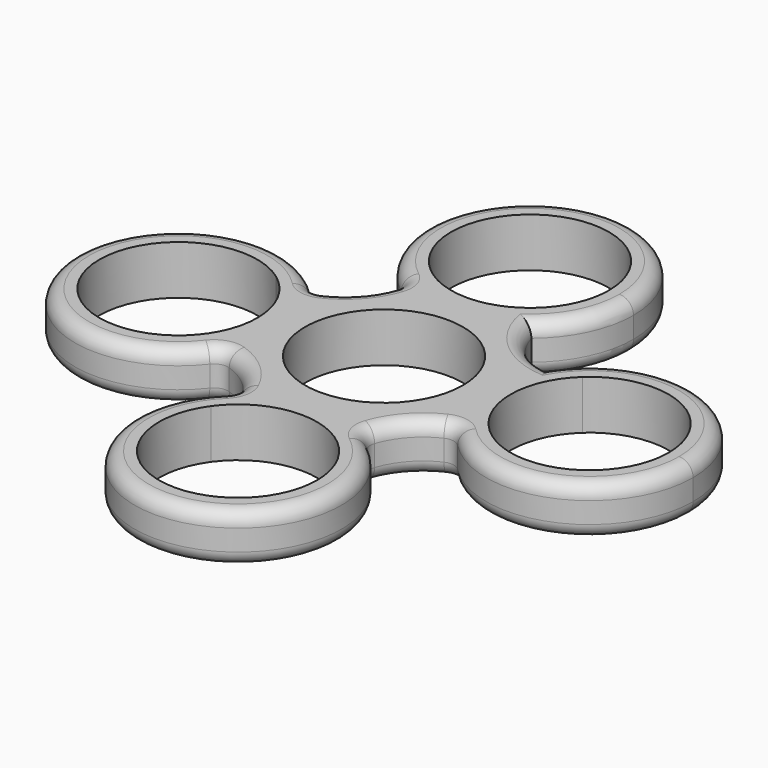
from build123d import *

# Parameters (mm, degrees)
F0_R     = 11.25
F1_DEPTH = 7
F2_R     = 2


with BuildPart() as f1:
    # F0 (on Top) → F1 (new body)
    with BuildSketch(Plane.XY):
        with BuildLine():
            ThreePointArc((-20.6818419333, 15.0335644628), (-21.5385463681, 19.9857387785), (-24.0090837029, 24.3623148626))
            ThreePointArc((-24.0090837029, 24.3623148626), (-26.4040491127, 23.960385675), (-28.8254223349, 24.1457450693))
            ThreePointArc((-28.8254223349, 24.1457450693), (-25.4035315724, 20.1491048046), (-24.1731995815, 15.0335644628))
            ThreePointArc((-24.1731995815, 15.0335644628), (-25.1151928743, 10.5271803553), (-27.7834213991, 6.7754599996))
            ThreePointArc((-27.7834213991, 6.7754599996), (-25.4145244015, 7.2193338549), (-23.0081257396, 7.0853843686))
            ThreePointArc((-23.0081257396, 7.0853843686), (-21.2753610709, 10.8927564753), (-20.6818419333, 15.0335644628))
        make_face()
        with BuildLine():
            ThreePointArc((-28.8254223349, 24.1457450693), (-26.4040491127, 23.960385675), (-24.0090837029, 24.3623148626))
            ThreePointArc((-24.0090837029, 24.3623148626), (-50.1398789796, 14.1809374616), (-23.0081257396, 7.0853843686))
            ThreePointArc((-23.0081257396, 7.0853843686), (-25.4145244015, 7.2193338549), (-27.7834213991, 6.7754599996))
            ThreePointArc((-27.7834213991, 6.7754599996), (-46.6530124471, 14.3599154428), (-28.8254223349, 24.1457450693))
        make_face()
        with BuildLine():
            ThreePointArc((0.2988637144, 33.2261356881), (-8.1772596841, 29.9235721685), (-16.9780667795, 32.2251777247))
            ThreePointArc((-16.9780667795, 32.2251777247), (-19.3767240664, 27.2950515881), (-24.0090837029, 24.3623148626))
            ThreePointArc((-24.0090837029, 24.3623148626), (-21.5385463681, 19.9857387785), (-20.6818419333, 15.0335644628))
            ThreePointArc((-20.6818419333, 15.0335644628), (-21.2753610709, 10.8927564753), (-23.0081257396, 7.0853843686))
            ThreePointArc((-23.0081257396, 7.0853843686), (-18.0779996029, 4.6867270817), (-15.1452628774, 0.0543674452))
            ThreePointArc((-15.1452628774, 0.0543674452), (-6.6691394789, 3.3569309648), (2.1316676166, 1.0553254086))
            ThreePointArc((2.1316676166, 1.0553254086), (4.5303249035, 5.9854515452), (9.16268454, 8.9181882707))
            ThreePointArc((9.16268454, 8.9181882707), (5.8601210204, 17.3943116693), (8.1617265766, 26.1951187647))
            ThreePointArc((8.1617265766, 26.1951187647), (3.23160044, 28.5937760516), (0.2988637144, 33.2261356881))
        make_face()
        with Locations((-7.4231995815, 16.6402515666)):
            Circle(F0_R, mode=Mode.SUBTRACT)
        with BuildLine():
            ThreePointArc((0.0822939211, 38.0424743201), (-8.3562376653, 33.410438701), (-17.2879911485, 37.0004733843))
            ThreePointArc((-17.2879911485, 37.0004733843), (-16.8441172933, 34.6315763866), (-16.9780667795, 32.2251777247))
            ThreePointArc((-16.9780667795, 32.2251777247), (-8.1772596841, 29.9235721685), (0.2988637144, 33.2261356881))
            ThreePointArc((0.2988637144, 33.2261356881), (-0.1030654731, 35.6211010979), (0.0822939211, 38.0424743201))
        make_face()
        with BuildLine():
            ThreePointArc((-17.2879911485, 37.0004733843), (-13.1322533674, 55.1156077709), (2.2201133147, 44.6402515666))
            ThreePointArc((2.2201133147, 44.6402515666), (1.6723217742, 41.1725096373), (0.0822939211, 38.0424743201))
            ThreePointArc((0.0822939211, 38.0424743201), (-0.1030654731, 35.6211010979), (0.2988637144, 33.2261356881))
            ThreePointArc((0.2988637144, 33.2261356881), (4.2897617966, 38.3240351653), (5.7114709628, 44.6402515666))
            ThreePointArc((5.7114709628, 44.6402515666), (-16.1059258277, 57.5722775241), (-16.9780667795, 32.2251777247))
            ThreePointArc((-16.9780667795, 32.2251777247), (-16.8441172933, 34.6315763866), (-17.2879911485, 37.0004733843))
        make_face()
        with BuildLine():
            ThreePointArc((35.3181580667, 18.2469386705), (24.717608406, 32.394777181), (8.1617265766, 26.1951187647))
            ThreePointArc((8.1617265766, 26.1951187647), (10.5681252385, 26.0611692784), (12.9370222362, 26.5050431337))
            ThreePointArc((12.9370222362, 26.5050431337), (25.083184526, 28.5549453777), (31.8268004185, 18.2469386705))
            ThreePointArc((31.8268004185, 18.2469386705), (25.6923407603, 8.2272706614), (13.979023172, 9.134758064))
            ThreePointArc((13.979023172, 9.134758064), (11.5576499498, 9.3201174583), (9.16268454, 8.9181882707))
            ThreePointArc((9.16268454, 8.9181882707), (25.5289747343, 4.3622854571), (35.3181580667, 18.2469386705))
        make_face()
        with BuildLine():
            ThreePointArc((12.9370222362, 26.5050431337), (10.5681252385, 26.0611692784), (8.1617265766, 26.1951187647))
            ThreePointArc((8.1617265766, 26.1951187647), (5.8601210204, 17.3943116693), (9.16268454, 8.9181882707))
            ThreePointArc((9.16268454, 8.9181882707), (11.5576499498, 9.3201174583), (13.979023172, 9.134758064))
            ThreePointArc((13.979023172, 9.134758064), (9.3469875529, 17.5732896505), (12.9370222362, 26.5050431337))
        make_face()
        with BuildLine():
            ThreePointArc((2.1316676166, 1.0553254086), (-6.6691394789, 3.3569309648), (-15.1452628774, 0.0543674452))
            ThreePointArc((-15.1452628774, 0.0543674452), (-14.7433336899, -2.3405979646), (-14.9286930841, -4.7619711868))
            ThreePointArc((-14.9286930841, -4.7619711868), (-6.4901614976, -0.1299355677), (2.4415919855, -3.719970251))
            ThreePointArc((2.4415919855, -3.719970251), (1.9977181303, -1.3510732534), (2.1316676166, 1.0553254086))
        make_face()
        with BuildLine():
            ThreePointArc((-14.9286930841, -4.7619711868), (-14.7433336899, -2.3405979646), (-15.1452628774, 0.0543674452))
            ThreePointArc((-15.1452628774, 0.0543674452), (-12.132728879, -24.6793969153), (8.9248451705, -11.3597484334))
            ThreePointArc((8.9248451705, -11.3597484334), (7.1155134799, -4.283709291), (2.1316676166, 1.0553254086))
            ThreePointArc((2.1316676166, 1.0553254086), (1.9977181303, -1.3510732534), (2.4415919855, -3.719970251))
            ThreePointArc((2.4415919855, -3.719970251), (4.6588437266, -7.2573817512), (5.4334875224, -11.3597484334))
            ThreePointArc((5.4334875224, -11.3597484334), (-9.284254407, -22.0619568929), (-14.9286930841, -4.7619711868))
        make_face()
    extrude(amount=F1_DEPTH)

    # F2
    f2_edges = [f1.edges().sort_by_distance(p)[0] for p in [
        (-9.882514, 59.356931, 7),
        (-16.978067, 32.225178, 3.5),
        (-24.009084, 24.362315, 3.5),
        (-19.376724, 27.295052, 0),
        (-19.376724, 27.295052, 7),
        (-23.008126, 7.085384, 3.5),
        (-15.145263, 0.054367, 3.5),
        (-18.078, 4.686727, 0),
        (-18.078, 4.686727, 7),
        (2.131668, 1.055325, 3.5),
        (9.162685, 8.918188, 3.5),
        (4.530325, 5.985452, 0),
        (4.530325, 5.985452, 7),
        (3.2316, 28.593776, 7),
        (3.2316, 28.593776, 0),
        (-50.139879, 14.180937, 0),
        (-50.139879, 14.180937, 7),
        (-4.963885, -26.076428, 0),
        (-4.963885, -26.076428, 7),
        (35.29348, 19.099566, 0),
        (35.29348, 19.099566, 7),
        (-9.882514, 59.356931, 0),
    ]]
    fillet(f2_edges, radius=F2_R)


solid = f1.part
